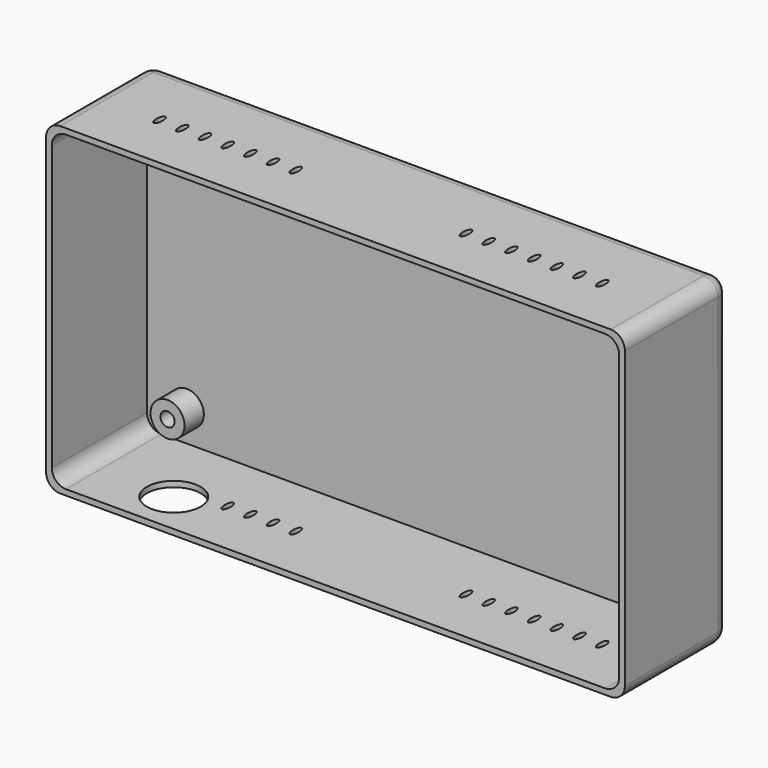
from build123d import *

# Parameters (mm, degrees)
F0_W           = 102
F0_H           = 57
F0_W_2         = 100
F0_H_2         = 55
F2_DEPTH       = 23
F1_W           = 100
F1_H           = 55
F1_R           = 3
F1_R_2         = 1.25
F3_DEPTH       = 2
F4_R           = 2.5
F5_T1_DEPTH    = 26.75
F5_S5_W        = 2.5
F5_S5_H        = 2.5
F5_T6_DEPTH    = 2.5
F5_S11_W       = 2.5
F5_S11_H       = 2.5
F5_T12_DEPTH   = 2.5
F5_S17_W       = 2.5
F5_S17_H       = 2.5
F5_T18_DEPTH   = 2.5
F5_S23_W       = 2.5
F5_S23_H       = 2.5
F5_T24_DEPTH   = 2.5
F6_R           = 2.5
F7_DEPTH       = 6.25
F9_DEPTH       = 57.001
F11_DEPTH      = 25
F11_DEPTH_BACK = 10
F10_R          = 4.75
F12_DEPTH      = 10


# Not quite as in the source:
# - a fillet or chamfer that OpenCascade refuses, or shapes differently, is made with other operations: its cross-section is extruded or revolved along the edge and cut away or added


with BuildPart() as f2:
    # F0 (on Front) → F2 (new body)
    with BuildSketch(Plane.XZ):
        Rectangle(F0_W, F0_H)
        Rectangle(F0_W_2, F0_H_2, mode=Mode.SUBTRACT)
    extrude(amount=F2_DEPTH)

    # F0 (on Front) + F1 (on face) → F3 (join)
    with BuildSketch(Plane.XZ):
        Rectangle(F0_W_2, F0_H_2)
    with BuildSketch(Plane.XZ):
        Rectangle(F1_W, F1_H)
        with Locations((-43, -22)):
            Circle(F1_R, mode=Mode.SUBTRACT)
        with Locations((43, -22)):
            Circle(F1_R, mode=Mode.SUBTRACT)
        with Locations((-43, 22)):
            Circle(F1_R, mode=Mode.SUBTRACT)
        with Locations((43, 22)):
            Circle(F1_R, mode=Mode.SUBTRACT)
        with Locations((43, 22)):
            Circle(F1_R)
        with Locations((43, 22)):
            Circle(F1_R_2, mode=Mode.SUBTRACT)
    extrude(amount=F3_DEPTH)

    # F4
    f4_edges = [f2.edges().sort_by_distance(p)[0] for p in [
        (0, 0, -28.5),
        (0, 0, 28.5),
        (-51, 0, 0),
        (51, 0, 0),
    ]]
    fillet(f4_edges, radius=F4_R)

    # F5: fillet of radius 2.5 on 4 edges, made by hand

    # F5_s2 → F5_t1 (cut)
    with BuildSketch(Plane.XZ.offset(2.5)):
        with BuildLine():
            ThreePointArc((-48.5, 28.5), (-50.267766953, 27.767766953), (-51, 26))
            Line((-51, 26), (-51, 28.5))
            Line((-51, 28.5), (-48.5, 28.5))
        make_face()
        with BuildLine():
            ThreePointArc((48.5, 28.5), (50.267766953, 27.767766953), (51, 26))
            Line((51, 26), (51, 28.5))
            Line((51, 28.5), (48.5, 28.5))
        make_face()
        with BuildLine():
            ThreePointArc((51, -26), (50.267766953, -27.767766953), (48.5, -28.5))
            Line((48.5, -28.5), (51, -28.5))
            Line((51, -28.5), (51, -26))
        make_face()
        with BuildLine():
            ThreePointArc((-51, -26), (-50.267766953, -27.767766953), (-48.5, -28.5))
            Line((-48.5, -28.5), (-51, -28.5))
            Line((-51, -28.5), (-51, -26))
        make_face()
    extrude(amount=F5_T1_DEPTH, mode=Mode.SUBTRACT)


with BuildPart() as f5_tool4:
    # F5_s5 → F5_t6 (new body)
    with BuildSketch(Plane.YZ.offset(-48.5)):
        with Locations((-1.25, -27.25)):
            Rectangle(F5_S5_W, F5_S5_H)
    extrude(amount=-F5_T6_DEPTH)

    # F5_s7 → F5_t8 (revolve, cut)
    with BuildSketch(Plane(origin=(-48.5, -2.5, -26), x_dir=(0, -0.7071067812, 0.7071067812), z_dir=(0, -0.7071067812, -0.7071067812))):
        with BuildLine():
            ThreePointArc((0, -2.5), (2.5, 0), (0, 2.5))
            Line((0, 2.5), (0, -2.5))
        make_face()
    revolve(axis=Axis((-48.5, -2.5, -26), (-1, 0, 0)), mode=Mode.SUBTRACT)


with BuildPart() as f2_1:
    add(f2.part)

    # F5_t3: cut F5_tool4
    add(f5_tool4.part, mode=Mode.SUBTRACT)


with BuildPart() as f5_tool10:
    # F5_s11 → F5_t12 (new body)
    with BuildSketch(Plane.YZ.offset(48.5)):
        with Locations((-1.25, -27.25)):
            Rectangle(F5_S11_W, F5_S11_H)
    extrude(amount=F5_T12_DEPTH)

    # F5_s13 → F5_t14 (revolve, cut)
    with BuildSketch(Plane(origin=(48.5, -2.5, -26), x_dir=(0, -0.7071067812, 0.7071067812), z_dir=(0, 0.7071067812, 0.7071067812))):
        with BuildLine():
            ThreePointArc((0, -2.5), (2.5, 0), (0, 2.5))
            Line((0, 2.5), (0, -2.5))
        make_face()
    revolve(axis=Axis((48.5, -2.5, -26), (1, 0, 0)), mode=Mode.SUBTRACT)


with BuildPart() as f2_2:
    add(f2_1.part)

    # F5_t9: cut F5_tool10
    add(f5_tool10.part, mode=Mode.SUBTRACT)


with BuildPart() as f5_tool16:
    # F5_s17 → F5_t18 (new body)
    with BuildSketch(Plane.XY.offset(26)):
        with Locations((49.75, -1.25)):
            Rectangle(F5_S17_W, F5_S17_H)
    extrude(amount=F5_T18_DEPTH)

    # F5_s19 → F5_t20 (revolve, cut)
    with BuildSketch(Plane(origin=(48.5, -2.5, 26), x_dir=(-0.7071067812, -0.7071067812, 0), z_dir=(-0.7071067812, 0.7071067812, 0))):
        with BuildLine():
            ThreePointArc((0, -2.5), (2.5, 0), (0, 2.5))
            Line((0, 2.5), (0, -2.5))
        make_face()
    revolve(axis=Axis((48.5, -2.5, 26), (0, 0, 1)), mode=Mode.SUBTRACT)


with BuildPart() as f2_3:
    add(f2_2.part)

    # F5_t15: cut F5_tool16
    add(f5_tool16.part, mode=Mode.SUBTRACT)


with BuildPart() as f5_tool22:
    # F5_s23 → F5_t24 (new body)
    with BuildSketch(Plane.XY.offset(26)):
        with Locations((-49.75, -1.25)):
            Rectangle(F5_S23_W, F5_S23_H)
    extrude(amount=F5_T24_DEPTH)

    # F5_s25 → F5_t26 (revolve, cut)
    with BuildSketch(Plane(origin=(-48.5, -2.5, 26), x_dir=(0.7071067812, -0.7071067812, 0), z_dir=(-0.7071067812, -0.7071067812, 0))):
        with BuildLine():
            ThreePointArc((0, -2.5), (2.5, 0), (0, 2.5))
            Line((0, 2.5), (0, -2.5))
        make_face()
    revolve(axis=Axis((-48.5, -2.5, 26), (0, 0, 1)), mode=Mode.SUBTRACT)


with BuildPart() as f2_4:
    add(f2_3.part)

    # F5_t21: cut F5_tool22
    add(f5_tool22.part, mode=Mode.SUBTRACT)

    # F6
    f6_edges = [f2_4.edges().sort_by_distance(p)[0] for p in [
        (-50, -12.5, -27.5),
        (-50, -12.5, 27.5),
        (50, -12.5, 27.5),
        (50, -12.5, -27.5),
    ]]
    fillet(f6_edges, radius=F6_R)

    # F1 (on face) → F7 (join)
    with BuildSketch(Plane.XZ):
        with Locations((-43, 22)):
            Circle(F1_R)
        with Locations((-43, 22)):
            Circle(F1_R_2, mode=Mode.SUBTRACT)
        with Locations((-43, -22)):
            Circle(F1_R)
        with Locations((-43, -22)):
            Circle(F1_R_2, mode=Mode.SUBTRACT)
        with Locations((43, -22)):
            Circle(F1_R)
        with Locations((43, -22)):
            Circle(F1_R_2, mode=Mode.SUBTRACT)
        with Locations((43, 22)):
            Circle(F1_R)
        with Locations((43, 22)):
            Circle(F1_R_2, mode=Mode.SUBTRACT)
    extrude(amount=F7_DEPTH)

    # F8 (on face) → F9 (cut, through all)
    with BuildSketch(Plane.XY.offset(28.5)):
        with BuildLine():
            add(Edge.make_bspline(
                [(14.5, -13), (14.5, -15.1650635095), (15.25, -14.0825317547), (16, -13), (15.25, -11.9174682453), (14.5, -10.8349364905), (14.5, -13)],
                knots=[4.7123889804, 4.7123889804, 4.7123889804, 6.8067840828, 6.8067840828, 8.9011791852, 8.9011791852, 10.9955742876, 10.9955742876, 10.9955742876], degree=2, weights=[1, 0.5, 1, 0.5, 1, 0.5, 1]))
        make_face()
        with BuildLine():
            add(Edge.make_bspline(
                [(18.5, -13), (18.5, -15.1650635095), (19.25, -14.0825317547), (20, -13), (19.25, -11.9174682453), (18.5, -10.8349364905), (18.5, -13)],
                knots=[4.7123889804, 4.7123889804, 4.7123889804, 6.8067840828, 6.8067840828, 8.9011791852, 8.9011791852, 10.9955742876, 10.9955742876, 10.9955742876], degree=2, weights=[1, 0.5, 1, 0.5, 1, 0.5, 1]))
        make_face()
        with BuildLine():
            add(Edge.make_bspline(
                [(22.5, -13), (22.5, -15.1650635095), (23.25, -14.0825317547), (24, -13), (23.25, -11.9174682453), (22.5, -10.8349364905), (22.5, -13)],
                knots=[4.7123889804, 4.7123889804, 4.7123889804, 6.8067840828, 6.8067840828, 8.9011791852, 8.9011791852, 10.9955742876, 10.9955742876, 10.9955742876], degree=2, weights=[1, 0.5, 1, 0.5, 1, 0.5, 1]))
        make_face()
        with BuildLine():
            add(Edge.make_bspline(
                [(26.5, -13), (26.5, -15.1650635095), (27.25, -14.0825317547), (28, -13), (27.25, -11.9174682453), (26.5, -10.8349364905), (26.5, -13)],
                knots=[4.7123889804, 4.7123889804, 4.7123889804, 6.8067840828, 6.8067840828, 8.9011791852, 8.9011791852, 10.9955742876, 10.9955742876, 10.9955742876], degree=2, weights=[1, 0.5, 1, 0.5, 1, 0.5, 1]))
        make_face()
        with BuildLine():
            add(Edge.make_bspline(
                [(30.5, -13), (30.5, -15.1650635095), (31.25, -14.0825317547), (32, -13), (31.25, -11.9174682453), (30.5, -10.8349364905), (30.5, -13)],
                knots=[4.7123889804, 4.7123889804, 4.7123889804, 6.8067840828, 6.8067840828, 8.9011791852, 8.9011791852, 10.9955742876, 10.9955742876, 10.9955742876], degree=2, weights=[1, 0.5, 1, 0.5, 1, 0.5, 1]))
        make_face()
        with BuildLine():
            add(Edge.make_bspline(
                [(34.5, -13), (34.5, -15.1650635095), (35.25, -14.0825317547), (36, -13), (35.25, -11.9174682453), (34.5, -10.8349364905), (34.5, -13)],
                knots=[4.7123889804, 4.7123889804, 4.7123889804, 6.8067840828, 6.8067840828, 8.9011791852, 8.9011791852, 10.9955742876, 10.9955742876, 10.9955742876], degree=2, weights=[1, 0.5, 1, 0.5, 1, 0.5, 1]))
        make_face()
        with BuildLine():
            add(Edge.make_bspline(
                [(38.5, -13), (38.5, -15.1650635095), (39.25, -14.0825317547), (40, -13), (39.25, -11.9174682453), (38.5, -10.8349364905), (38.5, -13)],
                knots=[4.7123889804, 4.7123889804, 4.7123889804, 6.8067840828, 6.8067840828, 8.9011791852, 8.9011791852, 10.9955742876, 10.9955742876, 10.9955742876], degree=2, weights=[1, 0.5, 1, 0.5, 1, 0.5, 1]))
        make_face()
        with BuildLine():
            add(Edge.make_bspline(
                [(-15.5, -13), (-15.5, -15.1650635095), (-14.75, -14.0825317547), (-14, -13), (-14.75, -11.9174682453), (-15.5, -10.8349364905), (-15.5, -13)],
                knots=[4.7123889804, 4.7123889804, 4.7123889804, 6.8067840828, 6.8067840828, 8.9011791852, 8.9011791852, 10.9955742876, 10.9955742876, 10.9955742876], degree=2, weights=[1, 0.5, 1, 0.5, 1, 0.5, 1]))
        make_face()
        with BuildLine():
            add(Edge.make_bspline(
                [(-19.5, -13), (-19.5, -15.1650635095), (-18.75, -14.0825317547), (-18, -13), (-18.75, -11.9174682453), (-19.5, -10.8349364905), (-19.5, -13)],
                knots=[4.7123889804, 4.7123889804, 4.7123889804, 6.8067840828, 6.8067840828, 8.9011791852, 8.9011791852, 10.9955742876, 10.9955742876, 10.9955742876], degree=2, weights=[1, 0.5, 1, 0.5, 1, 0.5, 1]))
        make_face()
        with BuildLine():
            add(Edge.make_bspline(
                [(-23.5, -13), (-23.5, -15.1650635095), (-22.75, -14.0825317547), (-22, -13), (-22.75, -11.9174682453), (-23.5, -10.8349364905), (-23.5, -13)],
                knots=[4.7123889804, 4.7123889804, 4.7123889804, 6.8067840828, 6.8067840828, 8.9011791852, 8.9011791852, 10.9955742876, 10.9955742876, 10.9955742876], degree=2, weights=[1, 0.5, 1, 0.5, 1, 0.5, 1]))
        make_face()
        with BuildLine():
            add(Edge.make_bspline(
                [(-27.5, -13), (-27.5, -15.1650635095), (-26.75, -14.0825317547), (-26, -13), (-26.75, -11.9174682453), (-27.5, -10.8349364905), (-27.5, -13)],
                knots=[4.7123889804, 4.7123889804, 4.7123889804, 6.8067840828, 6.8067840828, 8.9011791852, 8.9011791852, 10.9955742876, 10.9955742876, 10.9955742876], degree=2, weights=[1, 0.5, 1, 0.5, 1, 0.5, 1]))
        make_face()
    extrude(amount=-F9_DEPTH, mode=Mode.SUBTRACT)

    # F8 (on face) → F11 (cut, two sides)
    with BuildSketch(Plane.XY.offset(28.5)) as f11_sk:
        with BuildLine():
            add(Edge.make_bspline(
                [(-31.5, -13), (-31.5, -15.1650635095), (-30.75, -14.0825317547), (-30, -13), (-30.75, -11.9174682453), (-31.5, -10.8349364905), (-31.5, -13)],
                knots=[4.7123889804, 4.7123889804, 4.7123889804, 6.8067840828, 6.8067840828, 8.9011791852, 8.9011791852, 10.9955742876, 10.9955742876, 10.9955742876], degree=2, weights=[1, 0.5, 1, 0.5, 1, 0.5, 1]))
        make_face()
        with BuildLine():
            add(Edge.make_bspline(
                [(-35.5, -13), (-35.5, -15.1650635095), (-34.75, -14.0825317547), (-34, -13), (-34.75, -11.9174682453), (-35.5, -10.8349364905), (-35.5, -13)],
                knots=[4.7123889804, 4.7123889804, 4.7123889804, 6.8067840828, 6.8067840828, 8.9011791852, 8.9011791852, 10.9955742876, 10.9955742876, 10.9955742876], degree=2, weights=[1, 0.5, 1, 0.5, 1, 0.5, 1]))
        make_face()
        with BuildLine():
            add(Edge.make_bspline(
                [(-39.5, -13), (-39.5, -15.1650635095), (-38.75, -14.0825317547), (-38, -13), (-38.75, -11.9174682453), (-39.5, -10.8349364905), (-39.5, -13)],
                knots=[4.7123889804, 4.7123889804, 4.7123889804, 6.8067840828, 6.8067840828, 8.9011791852, 8.9011791852, 10.9955742876, 10.9955742876, 10.9955742876], degree=2, weights=[1, 0.5, 1, 0.5, 1, 0.5, 1]))
        make_face()
    extrude(amount=-F11_DEPTH, mode=Mode.SUBTRACT)
    extrude(f11_sk.sketch, amount=F11_DEPTH_BACK, mode=Mode.SUBTRACT)

    # F10 (on face) → F12 (cut)
    with BuildSketch(Plane(origin=(0, 0, -28.5), x_dir=(1, 0, 0), z_dir=(0, 0, -1))):
        with Locations((-34.5, 15.5)):
            Circle(F10_R)
    extrude(amount=-F12_DEPTH, mode=Mode.SUBTRACT)


solid = f2_4.part
